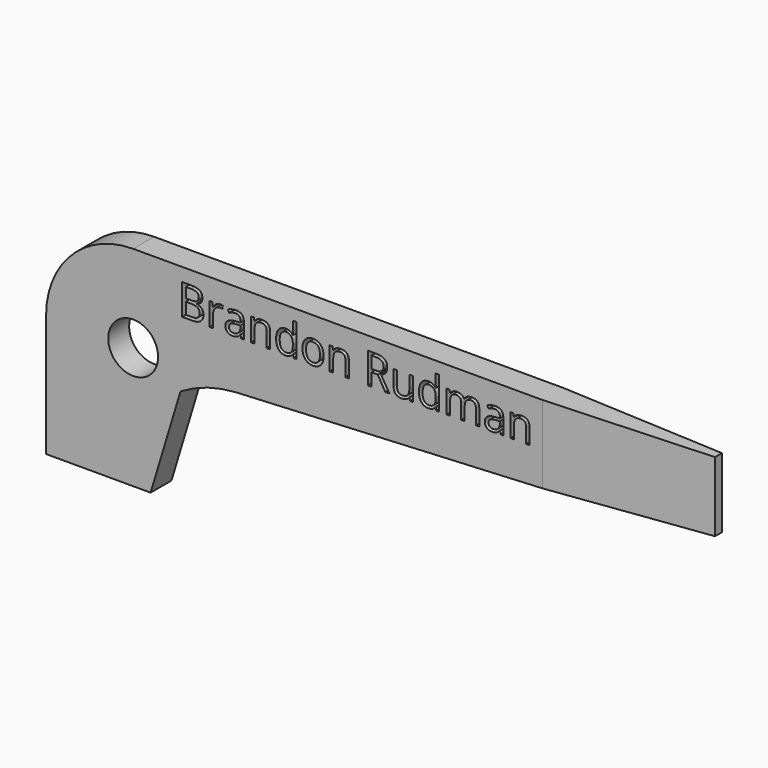
from build123d import *

# Parameters (mm, degrees)
F1_DEPTH     = 2.38125
F2_R         = 2.2716424119
F3_DEPTH     = 25.4
F5_DEPTH     = 25.4
F6_TEXT_SIZE = 3.9184427199
F7_DEPTH     = 1.27


# Not quite as in the source:
# - Text() gives the source's letters only with a copy of the font that has no kerning and outlines rounded to 1/6400 em; it was checked with that copy


with BuildPart() as f1:
    # F0 (on Front) → F1 (new body)
    with BuildSketch(Plane.XZ):
        with BuildLine():
            Line((60.325, 19.05), (7.9375, 19.05))
            ThreePointArc((7.9375, 19.05), (2.3248399243, 16.7251600757), (0, 11.1125))
            Line((0, 11.1125), (0, 0))
            Line((0, 0), (9.525, 0))
            Line((9.525, 0), (12.2510247766, 9.0160526091))
            ThreePointArc((12.2510247766, 9.0160526091), (14.7234940994, 10.1202730816), (17.3910038282, 10.5858901458))
            Line((17.3910038282, 10.5858901458), (60.325, 12.7))
            Line((60.325, 12.7), (60.325, 19.05))
        make_face()
    extrude(amount=F1_DEPTH)

    # F2 (on face) → F3 (cut)
    with BuildSketch(Plane.XZ.offset(2.38125)):
        with Locations((7.9375, 11.1125)):
            Circle(F2_R)
    extrude(amount=-F3_DEPTH, mode=Mode.SUBTRACT)

    # F4 (on face) → F5 (cut)
    with BuildSketch(Plane.XY.offset(19.05)):
        Polygon((60.325, -2.38125), (60.325, -1.5875), (45.24375, -2.38125), align=None)
        Polygon((60.325, 0), (45.24375, 0), (60.325, -0.79375), align=None)
    extrude(amount=-F5_DEPTH, mode=Mode.SUBTRACT)

    # F6 (on face) → F7 (cut)
    with BuildSketch(Plane.XZ.offset(2.38125)):
        with Locations((12.0212733746, 15.0401135907)):
            Text('Brandon Rudman', F6_TEXT_SIZE, font='Open Sans', text_align=(TextAlign.LEFT, TextAlign.BOTTOM))
    extrude(amount=-F7_DEPTH, mode=Mode.SUBTRACT)


solid = f1.part
